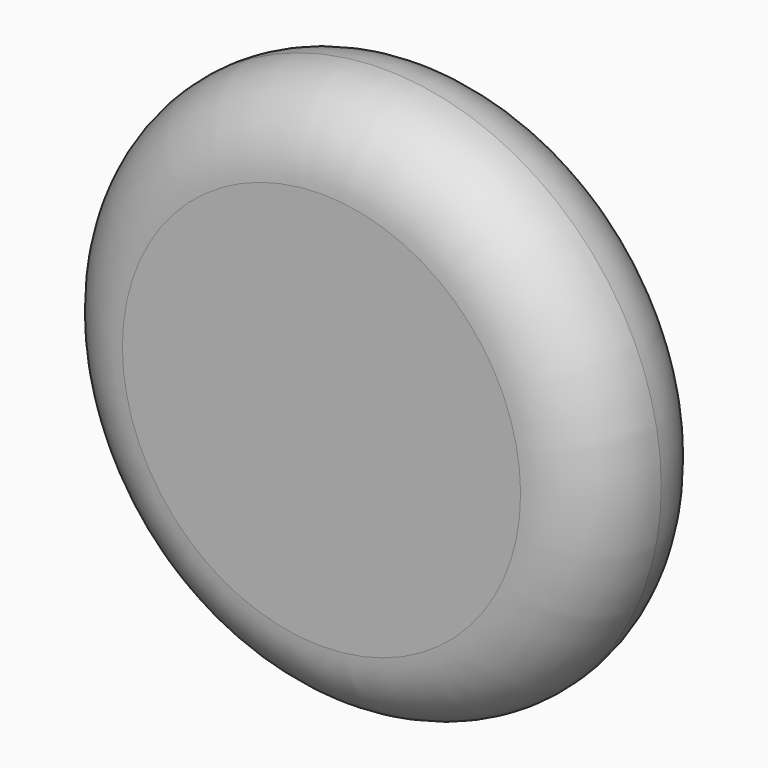
from build123d import *

# Parameters (mm, degrees)
F0_R     = 45.0575167081
F1_DEPTH = 25.4
F2_R     = 12.69999


# Not quite as in the source:
# - a fillet or chamfer is up to 0.001 mm smaller than in the source, because OpenCascade refuses the exact size


with BuildPart() as f1:
    # F0 (on Front) → F1 (new body)
    with BuildSketch(Plane.XZ):
        Circle(F0_R)
    extrude(amount=F1_DEPTH)

    # F2 (radius 12.7 in the source; OpenCascade refuses exactly that, so slightly less here)
    f2_edges = [f1.edges().sort_by_distance(p)[0] for p in [
        (-45.057517, -25.4, 0),
        (-45.057517, 0, 0),
    ]]
    fillet(f2_edges, radius=F2_R)


solid = f1.part
